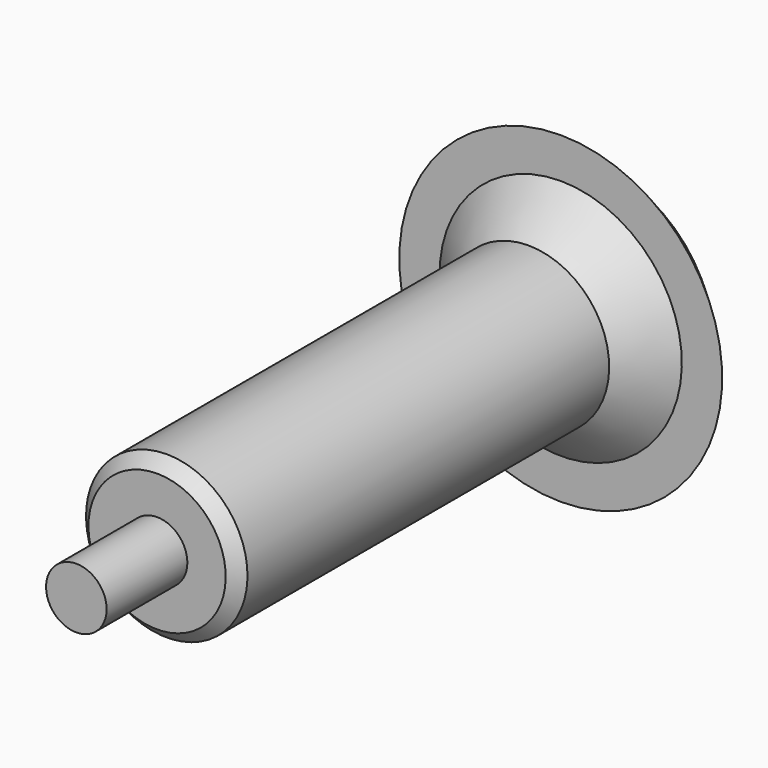
from build123d import *

# Parameters (mm, degrees)
F2_SIZE2 = 9.99999
F2_SIZE  = 9.99999
F3_SIZE2 = 10
F3_SIZE  = 10
F4_SIZE2 = 3
F4_SIZE  = 3


# Not quite as in the source:
# - a fillet or chamfer is up to 0.001 mm smaller than in the source, because OpenCascade refuses the exact size


with BuildPart() as f1:
    # F0 (on Right) → F1 (revolve)
    with BuildSketch(Plane.YZ):
        Polygon((-65.5954569578, 36.0077895969), (-65.5954569578, 28.5077895969), (84.4045430422, 28.5077895969), (94.4045430422, 28.5077895969), (94.4045430422, 68.5077895969), (84.4045430422, 68.5077895969), (84.4045430422, 48.5077895969), (-40.5954569578, 48.5077895969), (-40.5954569578, 36.0077895969), align=None)
    revolve(axis=Axis((0, 9.4045430422, 28.5077895969), (0, -1, 0)))

    # F2 (size 10 and 10 in the source; OpenCascade refuses exactly that, so slightly less here)
    f2_edges = [f1.edges().sort_by_distance(p)[0] for p in [
        (0, 94.404543, -11.49221),
    ]]
    chamfer(f2_edges, length=F2_SIZE, length2=F2_SIZE2)

    # F3
    f3_edges = [f1.edges().sort_by_distance(p)[0] for p in [
        (0, 84.404543, 8.50779),
    ]]
    chamfer(f3_edges, length=F3_SIZE, length2=F3_SIZE2)

    # F4
    f4_edges = [f1.edges().sort_by_distance(p)[0] for p in [
        (0, -40.595457, 8.50779),
    ]]
    chamfer(f4_edges, length=F4_SIZE, length2=F4_SIZE2)


solid = f1.part
